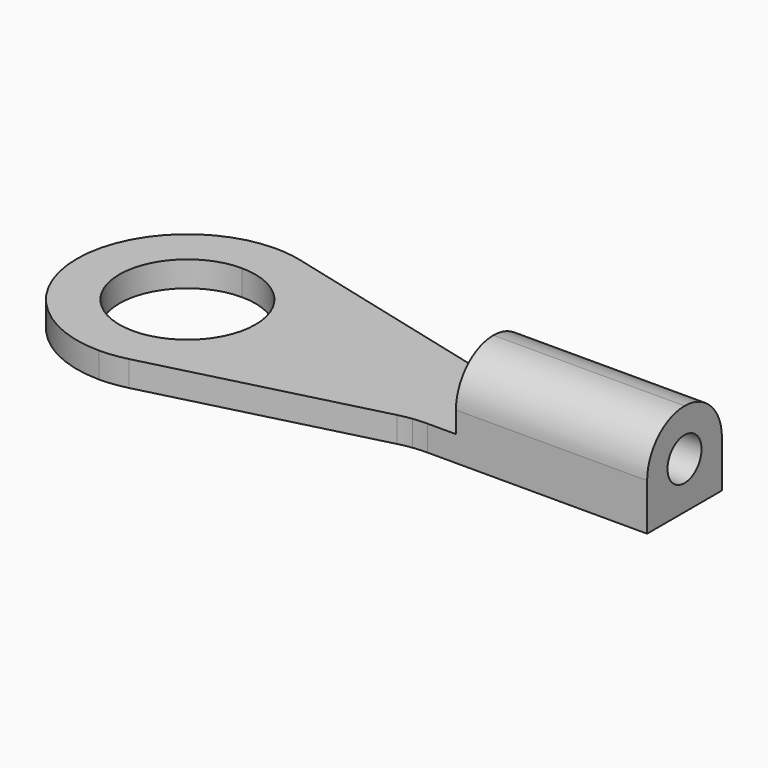
from build123d import *

# Parameters (mm, degrees)
F0_W     = 4.5
F0_H     = 1.1
F1_DEPTH = 0.6
F2_W     = 4.5
F2_H     = 2.2
F3_DEPTH = 1.6
F4_R     = 1.09999
F5_R     = 0.5
F6_DEPTH = 25


# Not quite as in the source:
# - a fillet or chamfer is up to 0.001 mm smaller than in the source, because OpenCascade refuses the exact size


with BuildPart() as f1:
    # F0 (on Top) → F1 (new body)
    with BuildSketch(Plane.XY):
        with Locations((12.05, 2.05)):
            Rectangle(F0_W, F0_H)
        with Locations((12.05, 3.15)):
            Rectangle(F0_W, F0_H)
        with BuildLine():
            Line((9.1267705413, 1.5), (9.8, 1.5))
            Line((9.8, 1.5), (9.8, 2.6))
            Line((9.8, 2.6), (8.8, 2.6))
            Line((8.8, 2.6), (8.8, 1.4793838437))
            ThreePointArc((8.8, 1.4793838437), (8.9630604221, 1.4948408423), (9.1267705413, 1.5))
        make_face()
        with BuildLine():
            Line((8.8, 2.6), (9.8, 2.6))
            Line((9.8, 2.6), (9.8, 3.7))
            Line((9.8, 3.7), (9.1267705413, 3.7))
            ThreePointArc((9.1267705413, 3.7), (8.9630604221, 3.7051591577), (8.8, 3.7206161563))
            Line((8.8, 3.7206161563), (8.8, 2.6))
        make_face()
        with BuildLine():
            Line((8.8, 1.4793838437), (8.8, 2.6))
            Line((8.8, 2.6), (8.8, 3.7206161563))
            ThreePointArc((8.8, 3.7206161563), (8.6407616767, 3.7458278477), (8.4833920771, 3.7808604342))
            Line((8.4833920771, 3.7808604342), (3.2433784641, 5.1191395658))
            ThreePointArc((3.2433784641, 5.1191395658), (2.9242199323, 5.1797056878), (2.6, 5.2))
            Line((2.6, 5.2), (2.6, 4.2))
            ThreePointArc((2.6, 4.2), (3.7313708499, 3.7313708499), (4.2, 2.6))
            ThreePointArc((4.2, 2.6), (3.7313708499, 1.4686291501), (2.6, 1))
            Line((2.6, 1), (2.6, 0))
            ThreePointArc((2.6, 0), (2.9242199323, 0.0202943122), (3.2433784641, 0.0808604342))
            Line((3.2433784641, 0.0808604342), (8.4833920771, 1.4191395658))
            ThreePointArc((8.4833920771, 1.4191395658), (8.6407616767, 1.4541721523), (8.8, 1.4793838437))
        make_face()
        with BuildLine():
            ThreePointArc((0, 2.6), (0.7615223689, 0.7615223689), (2.6, 0))
            Line((2.6, 0), (2.6, 1))
            ThreePointArc((2.6, 1), (1, 2.6), (2.6, 4.2))
            Line((2.6, 4.2), (2.6, 5.2))
            ThreePointArc((2.6, 5.2), (0.7615223689, 4.4384776311), (0, 2.6))
        make_face()
    extrude(amount=F1_DEPTH)

    # F2 (on face) → F3 (join)
    with BuildSketch(Plane.XY.offset(0.6)):
        with Locations((12.05, 2.6)):
            Rectangle(F2_W, F2_H)
    extrude(amount=F3_DEPTH)

    # F4 (radius 1.1 in the source; OpenCascade refuses exactly that, so slightly less here)
    f4_edges = [f1.edges().sort_by_distance(p)[0] for p in [
        (12.05, 1.5, 2.2),
        (12.05, 3.7, 2.2),
    ]]
    fillet(f4_edges, radius=F4_R)

    # F5 (on face) → F6 (cut)
    with BuildSketch(Plane.YZ.offset(14.3)):
        with Locations((2.6, 1.1)):
            Circle(F5_R)
    extrude(amount=-F6_DEPTH, mode=Mode.SUBTRACT)


solid = f1.part
